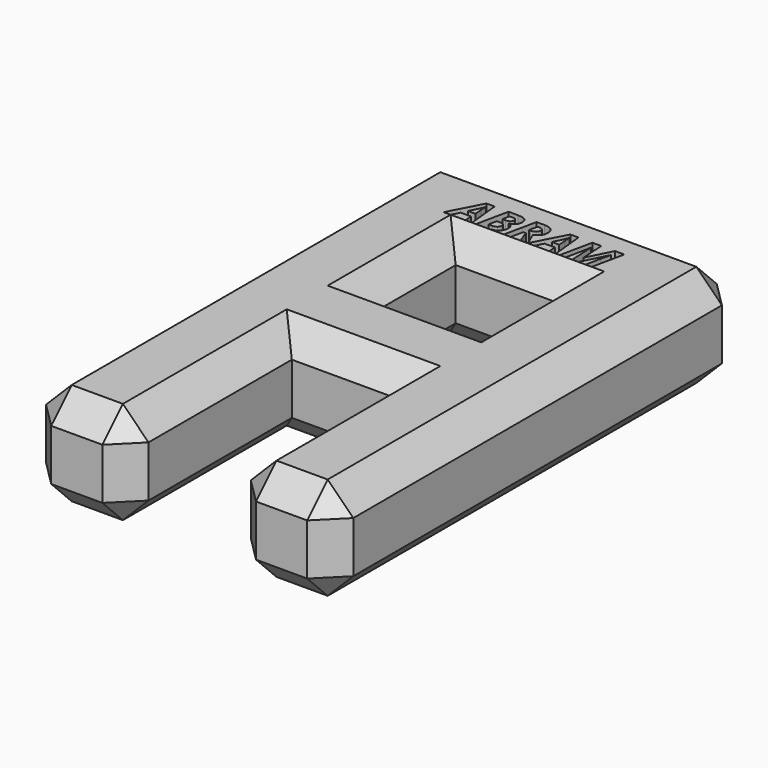
from build123d import *

# Parameters (mm, degrees)
F0_W     = 15.24
F0_H     = 25.4
F1_DEPTH = 5.08
F2_W     = 5.08
F2_H     = 5.08
F2_H_2   = 10.16
F3_DEPTH = 5.08
F4_SIZE  = 1.27
F6_DEPTH = 1.27


with BuildPart() as f1:
    # F0 (on Top) → F1 (new body)
    with BuildSketch(Plane.XY):
        Rectangle(F0_W, F0_H)
    extrude(amount=F1_DEPTH)

    # F2 (on face) → F3 (cut)
    with BuildSketch(Plane.XY.offset(5.08)):
        with Locations((0, 5.08)):
            Rectangle(F2_W, F2_H)
        with Locations((0, -7.62)):
            Rectangle(F2_W, F2_H_2)
    extrude(amount=-F3_DEPTH, mode=Mode.SUBTRACT)

    # F4
    f4_edges = [f1.edges().sort_by_distance(p)[0] for p in [
        (-7.62, 12.7, 2.54),
        (7.62, 12.7, 2.54),
        (0, 12.7, 0),
        (0, 12.7, 5.08),
        (-7.62, -12.7, 2.54),
        (-7.62, 0, 0),
        (-7.62, 0, 5.08),
        (7.62, -12.7, 2.54),
        (7.62, 0, 0),
        (7.62, 0, 5.08),
        (5.08, -12.7, 5.08),
        (2.54, -7.62, 5.08),
        (0, -2.54, 5.08),
        (-2.54, -7.62, 5.08),
        (-5.08, -12.7, 5.08),
        (0, 7.62, 5.08),
        (-2.54, 5.08, 5.08),
        (0, 2.54, 5.08),
        (2.54, 5.08, 5.08),
        (-5.08, -12.7, 0),
        (-2.54, -12.7, 2.54),
        (5.08, -12.7, 0),
        (2.54, -12.7, 2.54),
        (2.54, -7.62, 0),
        (0, -2.54, 0),
        (-2.54, -7.62, 0),
        (0, 7.62, 0),
        (-2.54, 5.08, 0),
        (0, 2.54, 0),
        (2.54, 5.08, 0),
    ]]
    chamfer(f4_edges, length=F4_SIZE)

    # F5 (on face) → F6 (cut)
    with BuildSketch(Plane.XY.offset(5.08)):
        Polygon((-3.6134711759, 9.2707446679), (-3.0962463422, 9.2707446679), (-3.0700001564, 8.89), (-2.7452473515, 8.89), (-2.9058740083, 10.4955666693), (-3.3139147093, 10.4955666693), (-4.1513430091, 8.89), (-3.8013938659, 8.89), align=None)
        with BuildLine():
            Line((-3.1410398325, 9.9377477349), (-3.1126939519, 9.5549033722))
            Line((-3.1126939519, 9.5549033722), (-3.4766410609, 9.5549033722))
            Line((-3.4766410609, 9.5549033722), (-3.2712209138, 9.9758921915))
            add(Edge.make_bspline(
                [(-3.151888256, 10.2537518113), (-3.2001812377, 10.1225208826), (-3.2712209138, 9.9758921915)],
                knots=[0, 0, 0, 1, 1, 1], degree=2))
            Line((-3.151888256, 10.2537518113), (-3.151888256, 10.2142075581))
            add(Edge.make_bspline(
                [(-3.1410398325, 9.9377477349), (-3.151888256, 10.0808769345), (-3.151888256, 10.2142075581)],
                knots=[0, 0, 0, 1, 1, 1], degree=2))
        make_face(mode=Mode.SUBTRACT)
        with BuildLine():
            add(Edge.make_bspline(
                [(-1.7485921915, 10.4889176355), (-1.4983785541, 10.4889176355), (-1.3704721422, 10.399680604)],
                knots=[0, 0, 0, 1, 1, 1], degree=2))
            Line((-1.7485921915, 10.4889176355), (-2.2147244503, 10.4889176355))
            Line((-2.2147244503, 10.4889176355), (-2.5524253736, 8.89))
            Line((-2.5524253736, 8.89), (-1.9816583209, 8.89))
            add(Edge.make_bspline(
                [(-1.5190255535, 9.025605293), (-1.686301244, 8.89), (-1.9816583209, 8.89)],
                knots=[0, 0, 0, 1, 1, 1], degree=2))
            add(Edge.make_bspline(
                [(-1.3517498631, 9.4117741726), (-1.3517498631, 9.161210586), (-1.5190255535, 9.025605293)],
                knots=[0, 0, 0, 1, 1, 1], degree=2))
            add(Edge.make_bspline(
                [(-1.4168404037, 9.6089705148), (-1.3517498631, 9.5318067287), (-1.3517498631, 9.4117741726)],
                knots=[0, 0, 0, 1, 1, 1], degree=2))
            add(Edge.make_bspline(
                [(-1.591115077, 9.7144801815), (-1.4819309443, 9.6861343009), (-1.4168404037, 9.6089705148)],
                knots=[0, 0, 0, 1, 1, 1], degree=2))
            Line((-1.591115077, 9.7144801815), (-1.591115077, 9.7211292152))
            add(Edge.make_bspline(
                [(-1.3332025585, 9.8626836437), (-1.4238393866, 9.7561241296), (-1.591115077, 9.7211292152)],
                knots=[0, 0, 0, 1, 1, 1], degree=2))
            add(Edge.make_bspline(
                [(-1.2425657304, 10.133369306), (-1.2425657304, 9.9692431578), (-1.3332025585, 9.8626836437)],
                knots=[0, 0, 0, 1, 1, 1], degree=2))
            add(Edge.make_bspline(
                [(-1.3704721422, 10.399680604), (-1.2425657304, 10.3104435725), (-1.2425657304, 10.133369306)],
                knots=[0, 0, 0, 1, 1, 1], degree=2))
        make_face()
        with BuildLine():
            Line((-1.9631110163, 9.1699593146), (-2.1597824348, 9.1699593146))
            Line((-2.1597824348, 9.1699593146), (-2.0701954542, 9.5867487442))
            Line((-2.0701954542, 9.5867487442), (-1.8899716454, 9.5867487442))
            add(Edge.make_bspline(
                [(-1.6898007354, 9.4093245286), (-1.6898007354, 9.5867487442), (-1.8899716454, 9.5867487442)],
                knots=[0, 0, 0, 1, 1, 1], degree=2))
            add(Edge.make_bspline(
                [(-1.7624151827, 9.2334750841), (-1.6898007354, 9.2969908536), (-1.6898007354, 9.4093245286)],
                knots=[0, 0, 0, 1, 1, 1], degree=2))
            add(Edge.make_bspline(
                [(-1.9631110163, 9.1699593146), (-1.8350296299, 9.1699593146), (-1.7624151827, 9.2334750841)],
                knots=[0, 0, 0, 1, 1, 1], degree=2))
        make_face(mode=Mode.SUBTRACT)
        with BuildLine():
            Line((-1.8514772396, 9.8555096862), (-2.0145535404, 9.8555096862))
            Line((-2.0145535404, 9.8555096862), (-1.9389645254, 10.2110580158))
            Line((-1.9389645254, 10.2110580158), (-1.7727386824, 10.2110580158))
            add(Edge.make_bspline(
                [(-1.5869156873, 10.0612797825), (-1.5869156873, 10.2110580158), (-1.7727386824, 10.2110580158)],
                knots=[0, 0, 0, 1, 1, 1], degree=2))
            add(Edge.make_bspline(
                [(-1.6530560754, 9.908701956), (-1.5869156873, 9.9618942258), (-1.5869156873, 10.0612797825)],
                knots=[0, 0, 0, 1, 1, 1], degree=2))
            add(Edge.make_bspline(
                [(-1.8514772396, 9.8555096862), (-1.7191964635, 9.8555096862), (-1.6530560754, 9.908701956)],
                knots=[0, 0, 0, 1, 1, 1], degree=2))
        make_face(mode=Mode.SUBTRACT)
        with BuildLine():
            Line((-0.8299756905, 8.89), (-0.6997946092, 9.5034608481))
            Line((-0.6997946092, 9.5034608481), (-0.5696135279, 9.5034608481))
            Line((-0.5696135279, 9.5034608481), (-0.3435463813, 8.89))
            Line((-0.3435463813, 8.89), (0.0078025585, 8.89))
            Line((0.0078025585, 8.89), (0.0143906787, 8.9026311305))
            Line((0.0143906787, 8.9026311305), (-0.2658576715, 9.5692512871))
            add(Edge.make_bspline(
                [(-0.0042706869, 9.753499511), (-0.0950824896, 9.6294425397), (-0.2658576715, 9.5692512871)],
                knots=[0, 0, 0, 1, 1, 1], degree=2))
            add(Edge.make_bspline(
                [(0.0865411157, 10.050431359), (0.0865411157, 9.8775564823), (-0.0042706869, 9.753499511)],
                knots=[0, 0, 0, 1, 1, 1], degree=2))
            add(Edge.make_bspline(
                [(-0.0436399656, 10.3772838588), (0.0865411157, 10.2656500821), (0.0865411157, 10.050431359)],
                knots=[0, 0, 0, 1, 1, 1], degree=2))
            add(Edge.make_bspline(
                [(-0.433133362, 10.4889176355), (-0.1738210468, 10.4889176355), (-0.0436399656, 10.3772838588)],
                knots=[0, 0, 0, 1, 1, 1], degree=2))
            Line((-0.433133362, 10.4889176355), (-0.8257763007, 10.4889176355))
            Line((-0.8257763007, 10.4889176355), (-1.163477224, 8.89))
            Line((-1.163477224, 8.89), (-0.8299756905, 8.89))
        make_face()
        with BuildLine():
            Line((-0.5566654096, 9.779220773), (-0.6420530005, 9.779220773))
            Line((-0.6420530005, 9.779220773), (-0.5500163758, 10.2110580158))
            Line((-0.5500163758, 10.2110580158), (-0.4691781238, 10.2110580158))
            add(Edge.make_bspline(
                [(-0.3055768993, 10.1662645255), (-0.3575443471, 10.2110580158), (-0.4691781238, 10.2110580158)],
                knots=[0, 0, 0, 1, 1, 1], degree=2))
            add(Edge.make_bspline(
                [(-0.2536094515, 10.0318840545), (-0.2536094515, 10.1214710351), (-0.3055768993, 10.1662645255)],
                knots=[0, 0, 0, 1, 1, 1], degree=2))
            add(Edge.make_bspline(
                [(-0.3335728307, 9.8415117205), (-0.2536094515, 9.903802668), (-0.2536094515, 10.0318840545)],
                knots=[0, 0, 0, 1, 1, 1], degree=2))
            add(Edge.make_bspline(
                [(-0.5566654096, 9.779220773), (-0.41353621, 9.779220773), (-0.3335728307, 9.8415117205)],
                knots=[0, 0, 0, 1, 1, 1], degree=2))
        make_face(mode=Mode.SUBTRACT)
        Polygon((0.0143906787, 8.9026311305), (0.0078025585, 8.89), (0.0197008294, 8.89), align=None)
        Polygon((0.0143906787, 8.9026311305), (0.0197008294, 8.89), (0.3577517018, 8.89), (0.5456743917, 9.2707446679), (1.0628992254, 9.2707446679), (1.0891454112, 8.89), (1.4138982161, 8.89), (1.2532715594, 10.4955666693), (0.8452308583, 10.4955666693), align=None)
        with BuildLine():
            Line((1.0181057351, 9.9377477349), (1.0464516157, 9.5549033722))
            Line((1.0464516157, 9.5549033722), (0.6825045067, 9.5549033722))
            Line((0.6825045067, 9.5549033722), (0.8879246538, 9.9758921915))
            add(Edge.make_bspline(
                [(1.0072573116, 10.2537518113), (0.9589643299, 10.1225208826), (0.8879246538, 9.9758921915)],
                knots=[0, 0, 0, 1, 1, 1], degree=2))
            Line((1.0072573116, 10.2537518113), (1.0072573116, 10.2142075581))
            add(Edge.make_bspline(
                [(1.0181057351, 9.9377477349), (1.0072573116, 10.0808769345), (1.0072573116, 10.2142075581)],
                knots=[0, 0, 0, 1, 1, 1], degree=2))
        make_face(mode=Mode.SUBTRACT)
        with BuildLine():
            Line((3.0677578672, 10.4889176355), (2.4651454425, 9.2934913622))
            Line((2.4651454425, 9.2934913622), (2.4605961036, 9.2934913622))
            Line((2.4605961036, 9.2934913622), (2.3864068852, 10.4889176355))
            Line((2.3864068852, 10.4889176355), (1.9444211173, 10.4889176355))
            Line((1.9444211173, 10.4889176355), (1.606720194, 8.89))
            Line((1.606720194, 8.89), (1.9073265081, 8.89))
            add(Edge.make_bspline(
                [(2.1118717823, 9.8765066348), (2.0823010797, 9.7200793678), (1.9073265081, 8.89)],
                knots=[0, 0, 0, 1, 1, 1], degree=2))
            add(Edge.make_bspline(
                [(2.1533407558, 10.1291699163), (2.1414424849, 10.0329339019), (2.1118717823, 9.8765066348)],
                knots=[0, 0, 0, 1, 1, 1], degree=2))
            Line((2.1533407558, 10.1291699163), (2.1578900947, 10.1291699163))
            Line((2.1578900947, 10.1291699163), (2.2243804319, 8.89))
            Line((2.2243804319, 8.89), (2.5316357797, 8.89))
            Line((2.5316357797, 8.89), (3.1541953055, 10.1291699163))
            Line((3.1541953055, 10.1291699163), (3.1594445427, 10.1291699163))
            add(Edge.make_bspline(
                [(3.0446612237, 9.6469399969), (3.1027527815, 9.9167507863), (3.1594445427, 10.1291699163)],
                knots=[0, 0, 0, 1, 1, 1], degree=2))
            Line((3.0446612237, 9.6469399969), (2.8861342618, 8.89))
            Line((2.8861342618, 8.89), (3.1923397621, 8.89))
            Line((3.1923397621, 8.89), (3.5303906345, 10.4889176355))
            Line((3.5303906345, 10.4889176355), (3.0677578672, 10.4889176355))
        make_face()
    extrude(amount=-F6_DEPTH, mode=Mode.SUBTRACT)


solid = f1.part
